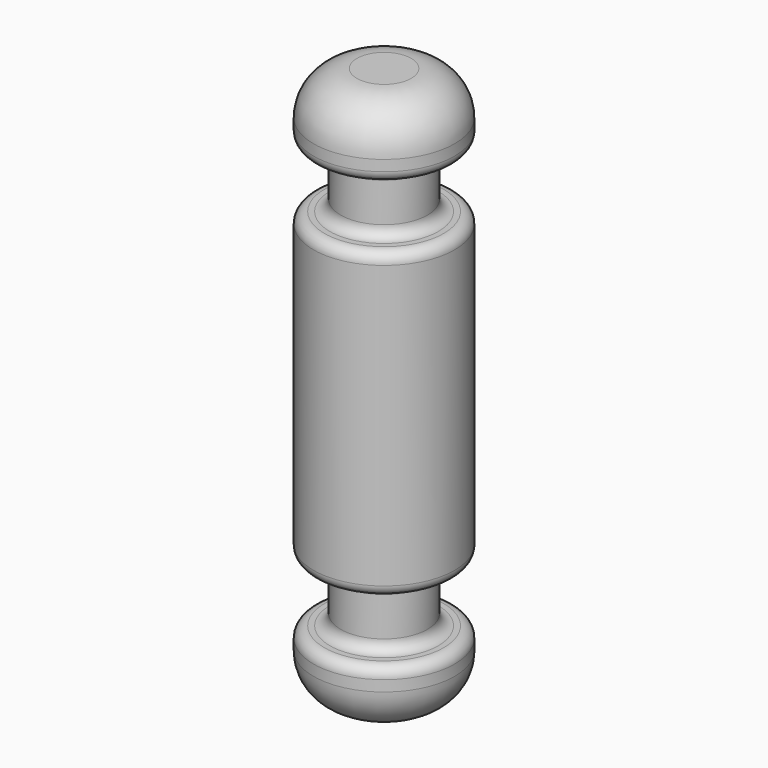
from build123d import *

# Parameters (mm, degrees)
F0_R          = 2
F1_DEPTH      = 9.8
F1_DEPTH_BACK = 9.8
F0_R_2        = 3.25
F2_DEPTH      = 7
F2_DEPTH_BACK = 7
F4_R          = 3.25
F5_DEPTH      = 3
F3_R          = 3.25
F6_DEPTH      = 3
F7_R          = 2
F8_R          = 0.5


with BuildPart() as f1:
    # F0 (on Top) → F1 (new body, two sides)
    with BuildSketch(Plane.XY) as f1_sk:
        Circle(F0_R)
    extrude(amount=F1_DEPTH)
    extrude(f1_sk.sketch, amount=-F1_DEPTH_BACK)

    # F0 (on Top) → F2 (join, two sides)
    with BuildSketch(Plane.XY) as f2_sk:
        Circle(F0_R_2)
        Circle(F0_R, mode=Mode.SUBTRACT)
    extrude(amount=F2_DEPTH)
    extrude(f2_sk.sketch, amount=-F2_DEPTH_BACK)

    # F4 (on face) → F5 (join)
    with BuildSketch(Plane.XY.offset(9.8)):
        Circle(F4_R)
    extrude(amount=F5_DEPTH)

    # F3 (on face) → F6 (join)
    with BuildSketch(Plane(origin=(0, 0, -9.8), x_dir=(1, 0, 0), z_dir=(0, 0, -1))):
        Circle(F3_R)
    extrude(amount=F6_DEPTH)

    # F7
    f7_edges = [f1.edges().sort_by_distance(p)[0] for p in [
        (-3.25, 0, 12.8),
        (-3.25, 0, -12.8),
    ]]
    fillet(f7_edges, radius=F7_R)

    # F8
    f8_edges = [f1.edges().sort_by_distance(p)[0] for p in [
        (-3.25, 0, 7),
        (-3.25, 0, -7),
        (-2, 0, -9.8),
        (-2, 0, -7),
        (-2, 0, 9.8),
        (-2, 0, 7),
        (-3.25, 0, 9.8),
        (-3.25, 0, -9.8),
    ]]
    fillet(f8_edges, radius=F8_R)


solid = f1.part
